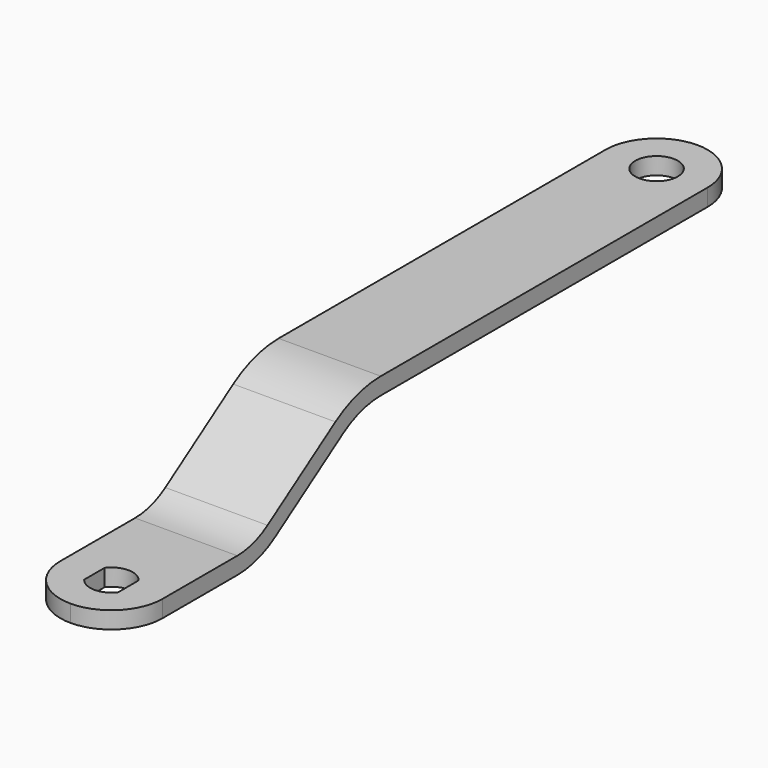
from build123d import *

# Parameters (mm, degrees)
F1_W     = 12
F1_H     = 2
F4_DEPTH = 2
F5_R     = 2.5
F6_DEPTH = 2
F7_R     = 5.99999
F8_R     = 5.99999


# Not quite as in the source:
# - a fillet or chamfer is up to 0.001 mm smaller than in the source, because OpenCascade refuses the exact size


with BuildPart() as f2:
    # F2: sweep along a path in F0
    with BuildLine(Plane.YZ) as f2_path:
        Line((0, 0), (16.9722436227, 0))
        ThreePointArc((16.9722436227, 0), (19.8700851096, 0.4290797351), (22.5192455849, 1.6794970566))
        Line((22.5192455849, 1.6794970566), (32.4807544151, 8.3205029434))
        ThreePointArc((32.4807544151, 8.3205029434), (35.1299148904, 9.5709202649), (38.0277563773, 10))
        Line((38.0277563773, 10), (92, 10))
    # F1 (on Front) → F2 (sweep)
    with BuildSketch(Plane.XZ):
        with Locations((0, 1)):
            Rectangle(F1_W, F1_H)
    sweep(path=f2_path.line)

    # F3 (on Top) → F4 (cut, through all)
    with BuildSketch(Plane.XY):
        with BuildLine():
            Line((2, 4.5), (2, 7.5))
            ThreePointArc((2, 7.5), (0, 8.5), (-2, 7.5))
            Line((-2, 7.5), (-2, 4.5))
            ThreePointArc((-2, 4.5), (0, 3.5), (2, 4.5))
        make_face()
    extrude(amount=F4_DEPTH, mode=Mode.SUBTRACT)

    # F5 (on face) → F6 (cut, through all)
    with BuildSketch(Plane.XY.offset(12)):
        with Locations((0, 86)):
            Circle(F5_R)
    extrude(amount=-F6_DEPTH, mode=Mode.SUBTRACT)

    # F7 (radius 6 in the source; OpenCascade refuses exactly that, so slightly less here)
    f7_edges = [f2.edges().sort_by_distance(p)[0] for p in [
        (6, 0, 1),
        (-6, 0, 1),
    ]]
    fillet(f7_edges, radius=F7_R)

    # F8 (radius 6 in the source; OpenCascade refuses exactly that, so slightly less here)
    f8_edges = [f2.edges().sort_by_distance(p)[0] for p in [
        (-6, 92, 11),
        (6, 92, 11),
    ]]
    fillet(f8_edges, radius=F8_R)


solid = f2.part
